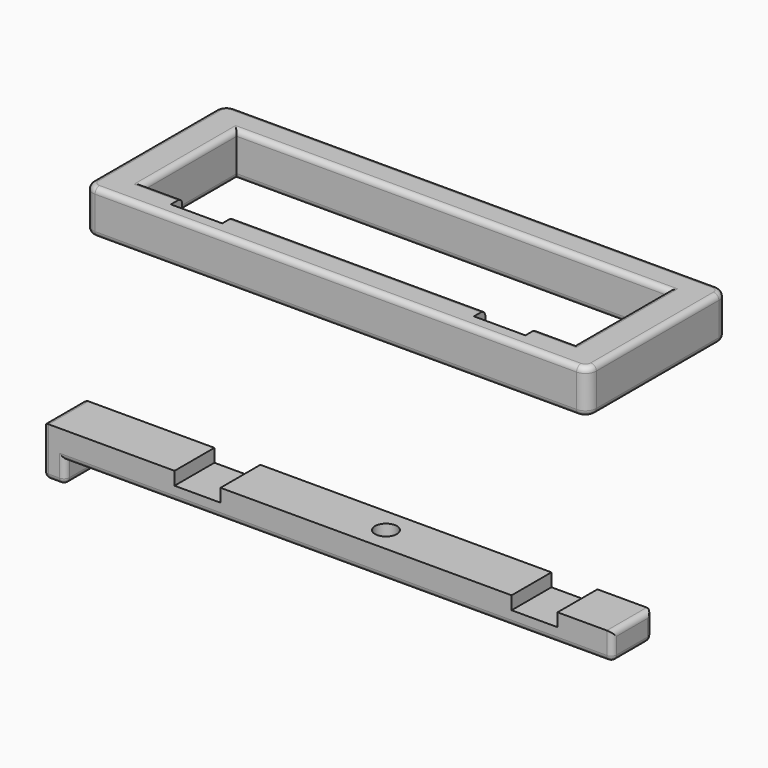
from build123d import *

# Parameters (mm, degrees)
F1_DEPTH       = 8
F2_W           = 10
F2_H           = 5
F3_DEPTH       = 9.1
F4_R           = 1
F6_R           = 1
F7_D           = 4
F7_START       = 0.2400659
F7_CSINK_D     = 8.4
F7_CSINK_ANGLE = 90
F8_R           = 1
F9_R           = 1
F10_R          = 1
F11_R          = 1
F12_R          = 1


# Not quite as in the source:
# - a feature names something its author has since deleted; it is built from what else it names


with BuildPart() as f1:
    # F0 (on Top) → F1 (new body)
    with BuildSketch(Plane.XY):
        with BuildLine():
            Line((-44, -16), (44, -16))
            ThreePointArc((44, -16), (45.4142135624, -15.4142135624), (46, -14))
            Line((46, -14), (46, 14))
            ThreePointArc((46, 14), (45.4142135624, 15.4142135624), (44, 16))
            Line((44, 16), (-44, 16))
            ThreePointArc((-44, 16), (-45.4142135624, 15.4142135624), (-46, 14))
            Line((-46, 14), (-46, -14))
            ThreePointArc((-46, -14), (-45.4142135624, -15.4142135624), (-44, -16))
        make_face()
        Polygon((39.4, 10.6), (39.4, -10.6), (32.4, -10.6), (32.4, -13.2), (23, -13.2), (23, -10.6), (-23, -10.6), (-23, -13.2), (-32.4, -13.2), (-32.4, -10.6), (-39.4, -10.6), (-39.4, 10.6), align=None, mode=Mode.SUBTRACT)
    extrude(amount=F1_DEPTH)

    # F4
    f4_edges = [f1.edges().sort_by_distance(p)[0] for p in [
        (0, -10.6, 0),
        (35.9, -10.6, 0),
        (35.9, -10.6, 8),
        (0, -10.6, 8),
        (-35.9, -10.6, 8),
        (-35.9, -10.6, 0),
    ]]
    fillet(f4_edges, radius=F4_R)

    # F9
    f9_edges = [f1.edges().sort_by_distance(p)[0] for p in [
        (0, 10.6, 0),
        (0, 10.6, 8),
    ]]
    fillet(f9_edges, radius=F9_R)

    # F10
    f10_edges = [f1.edges().sort_by_distance(p)[0] for p in [
        (46, 0, 0),
        (0, 16, 0),
        (45.414214, 15.414214, 0),
        (-46, 0, 0),
        (-45.414214, 15.414214, 0),
        (46, 0, 8),
        (0, 16, 8),
        (45.414214, 15.414214, 8),
        (-46, 0, 8),
        (-45.414214, 15.414214, 8),
    ]]
    fillet(f10_edges, radius=F10_R)

    # F11
    f11_edges = [f1.edges().sort_by_distance(p)[0] for p in [
        (39.4, 0, 8),
        (-39.4, 0, 8),
        (-39.4, 0, 0),
        (39.4, 0, 0),
    ]]
    fillet(f11_edges, radius=F11_R)


with BuildPart() as f3:
    # F2 (on Front) → F3 (new body)
    with BuildSketch(Plane.XZ):
        Polygon((-45, -37.3784252584), (-45, -42.3784252584), (45, -42.3784252584), (45, -37.3784252584), (35, -37.3784252584), (35, -39.7784252584), (26.6, -39.7784252584), (26.6, -37.3784252584), (-26.6, -37.3784252584), (-26.6, -39.7784252584), (-35, -39.7784252584), (-35, -37.3784252584), align=None)
        with Locations((-50, -39.8784252584)):
            Rectangle(F2_W, F2_H)
        Polygon((-55, -46.3784252584), (-55, -42.3784252584), (-55, -37.3784252584), (-59, -37.3784252584), (-59, -46.3784252584), align=None)
    extrude(amount=F3_DEPTH)

    # F6
    f6_edges = [f3.edges().sort_by_distance(p)[0] for p in [
        (-5, -9.1, -42.378425),
        (-5, 0, -42.378425),
    ]]
    fillet(f6_edges, radius=F6_R)

    # F7 (through all)
    # its depths count from where the whole tool has entered the part; down to there all is cleared
    with Locations(Plane(origin=(0, 0, -42.3784252584), x_dir=(1, 0, 0), z_dir=(0, 0, -1)).offset(-F7_START)):
        with Locations((0, 4.55)):
            CounterSinkHole(F7_D / 2, F7_CSINK_D / 2, counter_sink_angle=F7_CSINK_ANGLE)

    # F8
    f8_edges = [f3.edges().sort_by_distance(p)[0] for p in [
        (45, -4.55, -42.378425),
        (45, -4.55, -37.378425),
    ]]
    fillet(f8_edges, radius=F8_R)

    # F12
    f12_edges = [f3.edges().sort_by_distance(p)[0] for p in [
        (-55, -9.1, -43.878425),
        (-57, -9.1, -46.378425),
        (-59, -9.1, -41.878425),
        (-55, -4.55, -46.378425),
        (-59, -4.55, -46.378425),
        (-57, 0, -46.378425),
        (-55, 0, -43.878425),
        (-59, 0, -41.878425),
        (-59, -4.55, -37.378425),
    ]]
    fillet(f12_edges, radius=F12_R)


solid = Compound([f1.part, f3.part])
